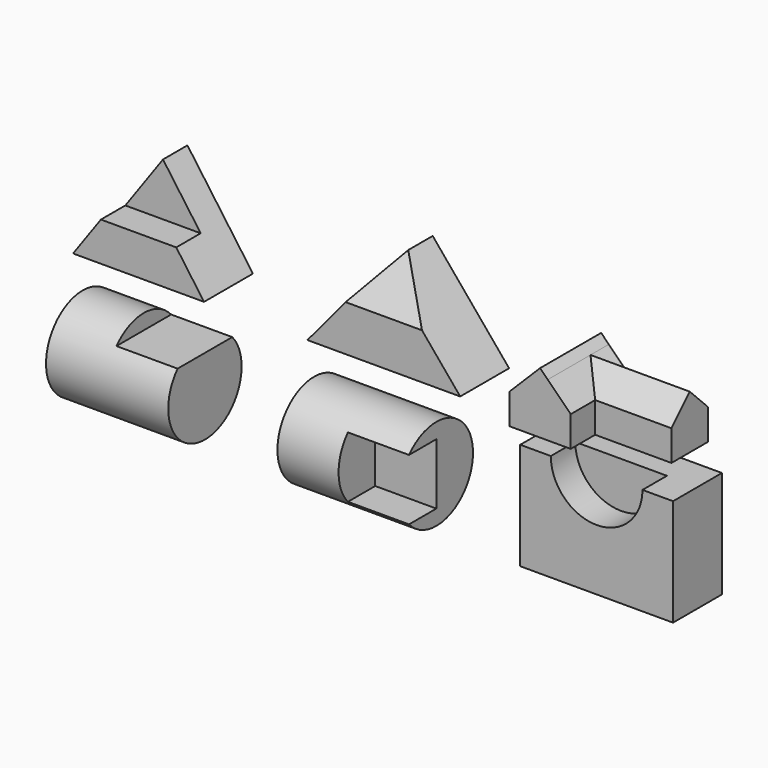
from build123d import *

# Parameters (mm, degrees)
F1_DEPTH  = 101.6
F2_DEPTH  = 50.8
F4_DEPTH  = 101.6
F8_DEPTH  = 76.2
F10_DEPTH = 127
F9_W      = 126.841150657
F9_H      = 50.8
F11_DEPTH = 76.2
F15_DEPTH = 203.2
F16_DEPTH = 101.6
F19_DEPTH = 203.2
F20_DEPTH = 101.6
F22_DEPTH = 101.6
F24_DEPTH = 50.8


with BuildPart() as f1:
    # F0 (on Front) → F1 (new body)
    with BuildSketch(Plane.XZ):
        Polygon((46.2219970567, 64.7107958794), (0, 0), (217.7142857143, 0), (171.4922886576, 64.7107958794), (108.8571428571, 64.7107958794), align=None)
    extrude(amount=F1_DEPTH)

    # F0 (on Front) → F2 (join)
    with BuildSketch(Plane.XZ):
        Polygon((46.2219970567, 64.7107958794), (0, 0), (217.7142857143, 0), (171.4922886576, 64.7107958794), (108.8571428571, 64.7107958794), align=None)
        Polygon((108.8571428571, 152.4), (46.2219970567, 64.7107958794), (108.8571428571, 64.7107958794), (171.4922886576, 64.7107958794), align=None)
    extrude(amount=F2_DEPTH)


with BuildPart() as f4:
    # F3 (on Front) → F4 (new body)
    with BuildSketch(Plane.XZ):
        Polygon((516.5779400596, 152.4), (389.5779400596, 0), (643.5779400596, 0), align=None)
    extrude(amount=F4_DEPTH)

    # F7 (on 3pt) → F8 (cut, symmetric)
    with BuildSketch(Plane.YZ.offset(516.5779400596)):
        Polygon((-50.8, 152.4), (-101.6, 152.4), (-101.6, 76.2), align=None)
    extrude(amount=F8_DEPTH, both=True, mode=Mode.SUBTRACT)


with BuildPart() as f10:
    # F9 (on Front) → F10 (new body)
    with BuildSketch(Plane.XZ):
        Polygon((745.8310411218, 50.8), (745.8310411218, 0), (847.5898904648, 0), (847.5898904648, 50.8), (809.3707534576, 88.9), (796.6310411218, 101.6), align=None)
    extrude(amount=F10_DEPTH)

    # F9 (on Front) → F11 (join)
    with BuildSketch(Plane.XZ):
        with Locations((911.0104657933, 25.4)):
            Rectangle(F9_W, F9_H)
    extrude(amount=F11_DEPTH)

    # F12 (on face) → F13 (join, up to the next surface of F10)
    with BuildSketch(Plane.YZ.offset(974.4310411218)):
        Polygon((-38.1, 88.9), (-76.2, 50.8), (0, 50.8), align=None)
    extrude(until=Until.NEXT, dir=(-1, 0, 0))


with BuildPart() as f15:
    # F14 (on Right) → F15 (new body)
    with BuildSketch(Plane.YZ):
        with BuildLine():
            ThreePointArc((-138.4216850644, -87.4777510762), (-108.8154016766, -209.4616848292), (-5.4255584359, -138.2777510762))
            ThreePointArc((-5.4255584359, -138.2777510762), (-10.441624683, -111.0879078355), (-24.8294318074, -87.4777510762))
            Line((-24.8294318074, -87.4777510762), (-81.6255584359, -87.4777510762))
            Line((-81.6255584359, -87.4777510762), (-138.4216850644, -87.4777510762))
        make_face()
    extrude(amount=F15_DEPTH)

    # F14 (on Right) → F16 (join)
    with BuildSketch(Plane.YZ):
        with BuildLine():
            Line((-81.6255584359, -87.4777510762), (-24.8294318074, -87.4777510762))
            ThreePointArc((-24.8294318074, -87.4777510762), (-81.6255584359, -62.0777510762), (-138.4216850644, -87.4777510762))
            Line((-138.4216850644, -87.4777510762), (-81.6255584359, -87.4777510762))
        make_face()
    extrude(amount=F16_DEPTH)


with BuildPart() as f19:
    # F18 (on offset) → F19 (new body)
    with BuildSketch(Plane.YZ.offset(386.08)):
        with BuildLine():
            ThreePointArc((-140.1055833345, -189.1506208658), (-56.1196134653, -209.5345546188), (-7.109456706, -138.3506208658))
            ThreePointArc((-7.109456706, -138.3506208658), (-56.1196134653, -67.1666871129), (-140.1055833345, -87.5506208658))
            Line((-140.1055833345, -87.5506208658), (-83.309456706, -87.5506208658))
            Line((-83.309456706, -87.5506208658), (-83.309456706, -189.1506208658))
            Line((-83.309456706, -189.1506208658), (-140.1055833345, -189.1506208658))
        make_face()
    extrude(amount=F19_DEPTH)

    # F18 (on offset) → F20 (join)
    with BuildSketch(Plane.YZ.offset(386.08)):
        with BuildLine():
            Line((-83.309456706, -87.5506208658), (-140.1055833345, -87.5506208658))
            ThreePointArc((-140.1055833345, -87.5506208658), (-159.509456706, -138.3506208658), (-140.1055833345, -189.1506208658))
            Line((-140.1055833345, -189.1506208658), (-83.309456706, -189.1506208658))
            Line((-83.309456706, -189.1506208658), (-83.309456706, -87.5506208658))
        make_face()
    extrude(amount=F20_DEPTH)


with BuildPart() as f22:
    # F21 (on Front) → F22 (new body)
    with BuildSketch(Plane.XZ):
        with BuildLine():
            Line((946.5842827101, -38.1610280335), (794.1842827101, -38.1610280335))
            ThreePointArc((794.1842827101, -38.1610280335), (870.3842827101, -114.3610280335), (946.5842827101, -38.1610280335))
        make_face()
        with BuildLine():
            Line((743.3842827101, -38.1610280335), (743.3842827101, -215.9610280335))
            Line((743.3842827101, -215.9610280335), (997.3842827101, -215.9610280335))
            Line((997.3842827101, -215.9610280335), (997.3842827101, -38.1610280335))
            Line((997.3842827101, -38.1610280335), (946.5842827101, -38.1610280335))
            ThreePointArc((946.5842827101, -38.1610280335), (870.3842827101, -114.3610280335), (794.1842827101, -38.1610280335))
            Line((794.1842827101, -38.1610280335), (743.3842827101, -38.1610280335))
        make_face()
    extrude(amount=F22_DEPTH)

    # F23 (on face) → F24 (cut)
    with BuildSketch(Plane.XZ.offset(101.6)):
        with BuildLine():
            Line((946.5842827101, -38.1610280335), (794.1842827101, -38.1610280335))
            ThreePointArc((794.1842827101, -38.1610280335), (870.3842827101, -114.3610280335), (946.5842827101, -38.1610280335))
        make_face()
    extrude(amount=-F24_DEPTH, mode=Mode.SUBTRACT)


solid = Compound([f1.part, f4.part, f10.part, f15.part, f19.part, f22.part])
